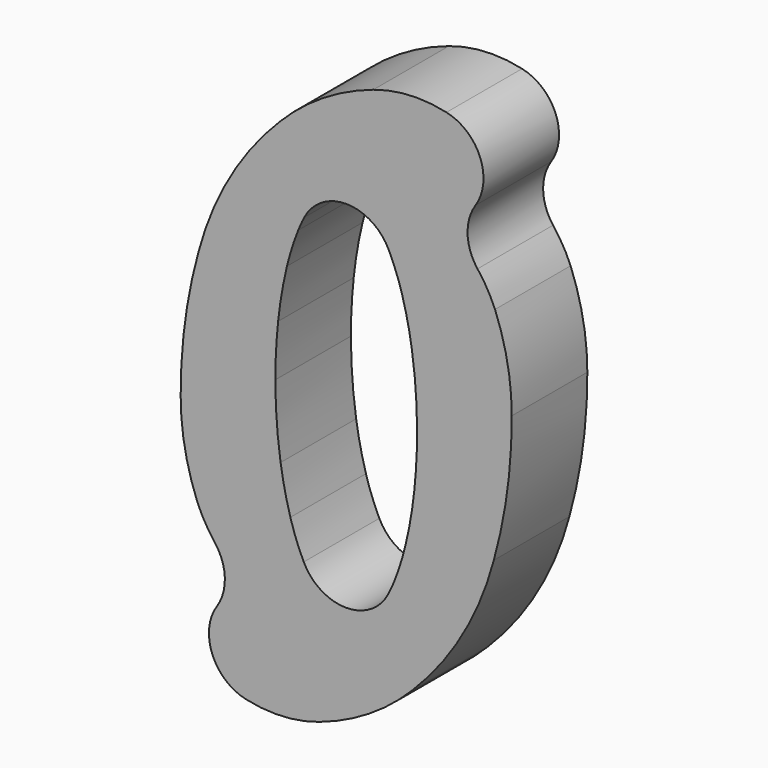
from build123d import *

# Parameters (mm, degrees)
F1_DEPTH = 12.7


# Not quite as in the source:
# - ends of sketch curves that miss each other by under 0.0002 mm in the source are joined


with BuildPart() as f1:
    # F0 (on Front) → F1 (new body)
    with BuildSketch(Plane.XZ):
        with BuildLine():
            ThreePointArc((303.2931532121, 303.0067577098), (301.4715319233, 294.1610584771), (300.8818774244, 285.1490106185))
            ThreePointArc((300.8818774244, 285.1490106185), (301.4449295055, 279.0945065847), (303.1390906491, 273.2546565343))
            ThreePointArc((303.1390906491, 273.2546565343), (304.1794047627, 271.163745604), (305.4871188741, 269.2287914427))
            ThreePointArc((305.4871188741, 269.2287914427), (306.8191261994, 265.559271793), (305.752743748, 261.8039536514))
            ThreePointArc((305.752743748, 261.8039536514), (305.1400456304, 255.9083712227), (309.6612562028, 252.0753703346))
            ThreePointArc((309.6612562028, 252.0753703346), (314.6118369552, 251.6558987634), (319.4911798503, 252.5919579373))
            ThreePointArc((319.4911798503, 252.5919579373), (326.238452414, 255.7664937708), (332.0491509461, 260.4397327714))
            ThreePointArc((332.0491509461, 260.4397327714), (338.7629233679, 269.1816350422), (342.9782332171, 279.3662684747))
            ThreePointArc((342.9782332171, 279.3662684747), (344.8007217874, 288.2183656036), (345.3891604556, 297.2369467464))
            ThreePointArc((345.3891604556, 297.2369467464), (344.8270625572, 303.274887915), (343.1402655074, 309.0996131302))
            ThreePointArc((343.1402655074, 309.0996131302), (342.0995588503, 311.1979660981), (340.7875354527, 313.1382632658))
            ThreePointArc((340.7875354527, 313.1382632658), (339.4517460358, 316.8098548296), (340.5182976713, 320.568494544))
            ThreePointArc((340.5182976713, 320.568494544), (341.1313810425, 326.4642550769), (336.610094213, 330.2975007104))
            ThreePointArc((336.610094213, 330.2975007104), (331.659512348, 330.7170042507), (326.7801614181, 329.7809489664))
            ThreePointArc((326.7801614181, 329.7809489664), (320.0328916386, 326.6063773725), (314.2221892806, 321.9331298991))
            ThreePointArc((314.2221892806, 321.9331298991), (307.5084491355, 313.1913079367), (303.2931532121, 303.0067577098))
        make_face()
        with BuildLine():
            ThreePointArc((315.1713123146, 305.1180818659), (315.8393495072, 307.515035294), (316.678097317, 309.857717846))
            ThreePointArc((316.678097317, 309.857717846), (317.0633180741, 310.7621499557), (317.4920222134, 311.6467997261))
            ThreePointArc((317.4920222134, 311.6467997261), (323.2069159103, 315.0891849126), (328.8450890708, 311.5225170196))
            ThreePointArc((328.8450890708, 311.5225170196), (329.8473834441, 309.2127575845), (330.6417253346, 306.8234892773))
            ThreePointArc((330.6417253346, 306.8234892773), (331.4003540176, 303.8138045335), (331.9581118177, 300.7605072271))
            ThreePointArc((331.9581118177, 300.7605072271), (332.4883254582, 295.994995702), (332.6606828218, 291.2031767897))
            ThreePointArc((332.6606828218, 291.2031767897), (332.5693501994, 287.6782798164), (332.2892894077, 284.1633395865))
            ThreePointArc((332.2892894077, 284.1633395865), (331.8093085942, 280.6893291587), (331.1000077041, 277.2547960368))
            ThreePointArc((331.1000077041, 277.2547960368), (330.4319997673, 274.8578337912), (329.5932507917, 272.5151498081))
            ThreePointArc((329.5932507917, 272.5151498081), (329.2080362587, 271.6107324514), (328.7793397252, 270.7260967499))
            ThreePointArc((328.7793397252, 270.7260967499), (323.064427394, 267.2836913001), (317.4262371292, 270.8503593804))
            ThreePointArc((317.4262371292, 270.8503593804), (316.4239511956, 273.1601221417), (315.6296075412, 275.5493890189))
            ThreePointArc((315.6296075412, 275.5493890189), (314.8709725785, 278.5590700417), (314.3132149314, 281.612365479))
            ThreePointArc((314.3132149314, 281.612365479), (313.7830008793, 286.3778788276), (313.6106433782, 291.1696996103))
            ThreePointArc((313.6106433782, 291.1696996103), (313.7020014012, 294.6945965951), (313.9820621923, 298.2095368135))
            ThreePointArc((313.9820621923, 298.2095368135), (314.4620178297, 301.6835485419), (315.1713123146, 305.1180818659))
        make_face(mode=Mode.SUBTRACT)
    extrude(amount=F1_DEPTH)


solid = f1.part
